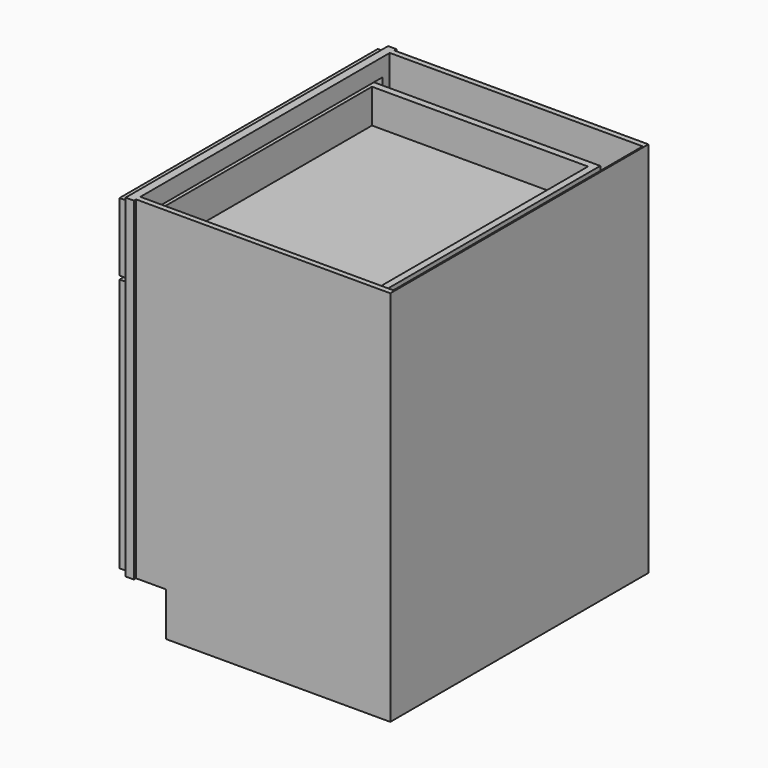
from build123d import *

# Parameters (mm, degrees)
F0_W          = 609.6
F0_H          = 876.3
F1_DEPTH      = 762
F2_W          = 88.9
F2_H          = 101.6
F3_DEPTH      = 762.001
F4_W          = 680.8032786885
F4_H          = 692.15
F5_DEPTH      = 19.05
F6_W          = 590.55
F6_H          = 6.35
F7_DEPTH      = 876.301
F8_W          = 587.375
F8_H          = 723.9
F9_DEPTH      = 733.425
F10_W         = 680.8032786885
F10_H         = 41.275
F11_DEPTH     = 19.05
F12_W         = 374.65
F12_H         = 590.5627
F12_W_2       = 260.35
F12_H_2       = 476.2627
F13_DEPTH     = 19.05
F14_W         = 6.35
F14_H         = 260.35
F15_DEPTH     = 476.2627
F16_SIZE      = 3.175
F17_W         = 749.3
F17_H         = 158.75
F17_W_2       = 635
F17_H_2       = 82.55
F18_DEPTH     = 19.05
F19_W         = 6.35
F19_H         = 635
F20_DEPTH     = 82.55
F21_SIZE      = 3.175
F22_W         = 504.825
F22_H         = 723.9
F23_DEPTH     = 101.6
F24_W         = 660.4
F24_H         = 95.25
F25_DEPTH     = 533.4
F26_T         = 15.875
F26_T3_DEPTH  = 37.249261314
F26_T5_DEPTH  = 37.249261314
F26_T7_DEPTH  = 37.249261314
F26_T9_DEPTH  = 37.249261314
F26_T11_DEPTH = 36.5125
F26_T13_DEPTH = 666.75
F26_T15_DEPTH = 114.3
F26_T17_DEPTH = 127
F26_T19_DEPTH = 692.15
F26_T21_DEPTH = 111.125
F26_T23_DEPTH = 36.5125


# Not quite as in the source:
# - a shell that OpenCascade refuses in one call is made with other operations: the cavity is built on its own and cut out


with BuildPart() as f1:
    # F0 (on Front) → F1 (new body)
    with BuildSketch(Plane.XZ):
        Rectangle(F0_W, F0_H)
    extrude(amount=-F1_DEPTH)

    # F2 (on face) → F3 (cut, through all)
    with BuildSketch(Plane.XZ):
        with Locations((-260.35, -387.35)):
            Rectangle(F2_W, F2_H)
    extrude(amount=-F3_DEPTH, mode=Mode.SUBTRACT)

    # F4 (on face) → F5 (cut)
    with BuildSketch(Plane(origin=(-304.8, 0, 0), x_dir=(0, -1, 0), z_dir=(-1, 0, 0))):
        with Locations((-381, 50.8)):
            Rectangle(F4_W, F4_H)
    extrude(amount=-F5_DEPTH, mode=Mode.SUBTRACT)

    # F6 (on face) → F7 (cut, through all)
    with BuildSketch(Plane.XY.offset(438.15)):
        with Locations((9.525, 758.825)):
            Rectangle(F6_W, F6_H)
        with Locations((9.525, 3.175)):
            Rectangle(F6_W, F6_H)
    extrude(amount=-F7_DEPTH, mode=Mode.SUBTRACT)

    # F8 (on face) → F9 (cut, through all)
    with BuildSketch(Plane.XY.offset(438.15)):
        with Locations((7.9375, 381)):
            Rectangle(F8_W, F8_H)
    extrude(amount=-F9_DEPTH, mode=Mode.SUBTRACT)

    # F10 (on face) → F11 (join, through all)
    with BuildSketch(Plane(origin=(-304.8, 0, 0), x_dir=(0, -1, 0), z_dir=(-1, 0, 0))):
        with Locations((-381, 265.1125)):
            Rectangle(F10_W, F10_H)
    extrude(amount=-F11_DEPTH)

    # F22 (on face) → F23 (cut)
    with BuildSketch(Plane(origin=(0, 0, -438.15), x_dir=(1, 0, 0), z_dir=(0, 0, -1))):
        with Locations((49.2125, -381)):
            Rectangle(F22_W, F22_H)
    extrude(amount=-F23_DEPTH, mode=Mode.SUBTRACT)


with BuildPart() as f13:
    # F12 (on face) → F13 (new body)
    with BuildSketch(Plane(origin=(-304.8, 0, 0), x_dir=(0, -1, 0), z_dir=(-1, 0, 0))):
        with Locations((-568.325, -33.33115)):
            Rectangle(F12_W, F12_H)
        with Locations((-568.325, -33.33115)):
            Rectangle(F12_W_2, F12_H_2, mode=Mode.SUBTRACT)
    extrude(amount=F13_DEPTH)

    # F14 (on face) → F15 (join, through all)
    with BuildSketch(Plane.XY.offset(-271.4625)):
        with Locations((-312.7375, 568.325)):
            Rectangle(F14_W, F14_H)
    extrude(amount=F15_DEPTH)

    # F16
    f16_edges = [f13.edges().sort_by_distance(p)[0] for p in [
        (-323.85, 698.5, -33.33115),
        (-323.85, 568.325, -271.4625),
        (-323.85, 438.15, -33.33115),
        (-323.85, 568.325, 204.8002),
    ]]
    chamfer(f16_edges, length=F16_SIZE)


with BuildPart() as f18:
    # F17 (on face) → F18 (new body)
    with BuildSketch(Plane(origin=(-304.8, 0, 0), x_dir=(0, -1, 0), z_dir=(-1, 0, 0))):
        with Locations((-381, 349.25)):
            Rectangle(F17_W, F17_H)
        with Locations((-381, 349.25)):
            Rectangle(F17_W_2, F17_H_2, mode=Mode.SUBTRACT)
    extrude(amount=F18_DEPTH)

    # F19 (on face) → F20 (join, through all)
    with BuildSketch(Plane.XY.offset(307.975)):
        with Locations((-312.7375, 381)):
            Rectangle(F19_W, F19_H)
    extrude(amount=F20_DEPTH)

    # F21
    f21_edges = [f18.edges().sort_by_distance(p)[0] for p in [
        (-323.85, 381, 307.975),
        (-323.85, 698.5, 349.25),
        (-323.85, 381, 390.525),
        (-323.85, 63.5, 349.25),
    ]]
    chamfer(f21_edges, length=F21_SIZE)

    # F24 (on face) → F25 (join)
    with BuildSketch(Plane.YZ.offset(-304.8)):
        with Locations((381, 339.725)):
            Rectangle(F24_W, F24_H)
    extrude(amount=F25_DEPTH)

    # F26: shell of thickness 15.875, made by hand


with BuildPart() as f26_core1:
    # F26_t2: copy of F18
    add(f18.part)

    # the walls: a layer under each face that stays
    f26_faces = [f26_core1.faces().sort_by_distance(p)[0] for p in [
        (-323.85, 630.7666666667, 296.3333333333),
        (-322.2625, 381, 306.3875),
        (-322.2625, 61.9125, 349.25),
        (-322.2625, 700.0875, 349.25),
        (-322.2625, 381, 392.1125),
        (-314.325, 381, 428.625),
        (-314.325, 755.65, 349.25),
        (-314.325, 381, 269.875),
        (-314.325, 6.35, 349.25),
        (-318.29375, 381, 307.975),
        (-318.29375, 63.5, 349.25),
        (-318.29375, 698.5, 349.25),
        (-318.29375, 381, 390.525),
        (-304.8, 630.7666666667, 402.1666666667),
        (-315.9125, 381, 349.25),
        (-38.1, 711.2, 339.725),
        (-38.1, 381, 292.1),
        (-38.1, 50.8, 339.725),
        (-307.18125, 63.5, 349.25),
        (-307.18125, 381, 390.525),
        (-307.18125, 698.5, 349.25),
        (-304.8, 381, 347.6625),
        (228.6, 381, 339.725),
        (-307.18125, 381, 307.975),
        (-309.5625, 381, 349.25),
    ]]
    thicken(f26_faces, amount=-F26_T, mode=Mode.SUBTRACT)

    # F26_s4 → F26_t3 (cut)
    with BuildSketch(Plane(origin=(4.5928978099, 4.5928978099, 4.5928978099), x_dir=(-0.7071067812, 0.7071067812, 0), z_dir=(0.5773502692, 0.5773502692, 0.5773502692))):
        Polygon((271.8908726623, 356.5892701441), (263.7152476623, 342.7036353262), (255.7777476623, 347.2863530879), (255.7777476623, 356.4517886113), align=None)
    extrude(amount=F26_T3_DEPTH, mode=Mode.SUBTRACT)

    # F26_s6 → F26_t5 (cut)
    with BuildSketch(Plane(origin=(-249.4071021901, 249.40710219, -249.4071021901), x_dir=(0.7071067812, 0.7071067812, 0), z_dir=(0.5773502692, -0.5773502692, 0.5773502692))):
        Polygon((266.9244946018, 667.6744674776), (275.1001196018, 653.7888326596), (283.0376196018, 658.3715504213), (283.0376196018, 667.5369859447), align=None)
    extrude(amount=F26_T5_DEPTH, mode=Mode.SUBTRACT)

    # F26_s8 → F26_t7 (cut)
    with BuildSketch(Plane(origin=(-228.2404355234, -228.2404355234, 228.2404355234), x_dir=(-0.7071067812, 0.7071067812, 0), z_dir=(0.5773502692, 0.5773502692, -0.5773502692))):
        Polygon((271.8908726623, 213.7335916339), (255.7777476623, 213.8710731668), (255.7777476623, 223.0365086901), (263.7152476623, 227.6192264518), align=None)
    extrude(amount=F26_T7_DEPTH, mode=Mode.SUBTRACT)

    # F26_s10 → F26_t9 (cut)
    with BuildSketch(Plane(origin=(-482.2404355234, 482.2404355234, 482.2404355234), x_dir=(0.7071067812, 0.7071067812, 0), z_dir=(0.5773502692, -0.5773502692, -0.5773502692))):
        Polygon((266.9244946018, -97.3516056996), (283.0376196018, -97.2141241667), (283.0376196018, -88.0486886433), (275.1001196018, -83.4659708816), align=None)
    extrude(amount=F26_T9_DEPTH, mode=Mode.SUBTRACT)

    # F26_s12 → F26_t11 (cut)
    with BuildSketch(Plane.YZ.offset(-336.55)):
        Polygon((698.34125, 308.13375), (698.5, 292.1), (714.375, 292.1), (714.375, 307.975), align=None)
        Polygon((63.65875, 308.13375), (63.5, 292.1), (47.625, 292.1), (47.625, 307.975), align=None)
        Polygon((63.65875, 390.36625), (47.625, 390.525), (47.625, 406.4), (63.5, 406.4), align=None)
        Polygon((698.34125, 390.36625), (714.375, 390.525), (714.375, 406.4), (698.5, 406.4), align=None)
    extrude(amount=F26_T11_DEPTH, mode=Mode.SUBTRACT)

    # F26_s14 → F26_t13 (cut)
    with BuildSketch(Plane.XZ.offset(-714.375)):
        Polygon((-316.07125, 308.13375), (-315.9125, 292.1), (-300.0375, 292.1), (-300.0375, 307.975), align=None)
        Polygon((-316.07125, 390.36625), (-315.9125, 406.4), (-300.0375, 406.4), (-300.0375, 390.525), align=None)
        Polygon((-309.40375, 390.36625), (-309.5625, 406.4), (-325.4375, 406.4), (-325.4375, 390.525), align=None)
        Polygon((-304.95875, 308.13375), (-288.925, 307.975), (-288.925, 292.1), (-304.8, 292.1), align=None)
        Polygon((-309.40375, 308.13375), (-309.5625, 292.1), (-325.4375, 292.1), (-325.4375, 307.975), align=None)
    extrude(amount=F26_T13_DEPTH, mode=Mode.SUBTRACT)

    # F26_s16 → F26_t15 (cut)
    with BuildSketch(Plane.XY.offset(292.1)):
        Polygon((-316.07125, 63.65875), (-315.9125, 47.625), (-300.0375, 47.625), (-300.0375, 63.5), align=None)
        Polygon((-316.07125, 698.34125), (-315.9125, 714.375), (-300.0375, 714.375), (-300.0375, 698.5), align=None)
        Polygon((-309.40375, 63.65875), (-309.5625, 47.625), (-325.4375, 47.625), (-325.4375, 63.5), align=None)
        Polygon((-309.40375, 698.34125), (-309.5625, 714.375), (-325.4375, 714.375), (-325.4375, 698.5), align=None)
    extrude(amount=F26_T15_DEPTH, mode=Mode.SUBTRACT)

    # F26_s18 → F26_t17 (cut)
    with BuildSketch(Plane.XY.offset(276.225)):
        Polygon((-304.64125, 711.35875), (-320.675, 711.2), (-320.675, 695.325), (-304.8, 695.325), align=None)
        Polygon((-304.64125, 50.64125), (-320.675, 50.8), (-320.675, 66.675), (-304.8, 66.675), align=None)
    extrude(amount=F26_T17_DEPTH, mode=Mode.SUBTRACT)

    # F26_s20 → F26_t19 (cut)
    with BuildSketch(Plane.XZ.offset(-727.075)):
        Polygon((-304.64125, 291.94125), (-320.675, 292.1), (-320.675, 307.975), (-304.8, 307.975), align=None)
    extrude(amount=F26_T19_DEPTH, mode=Mode.SUBTRACT)

    # F26_s22 → F26_t21 (cut)
    with BuildSketch(Plane.XY.offset(292.1)):
        Polygon((-304.95875, 63.65875), (-304.8, 47.625), (-288.925, 47.625), (-288.925, 63.5), align=None)
        Polygon((-304.95875, 698.34125), (-304.8, 714.375), (-288.925, 714.375), (-288.925, 698.5), align=None)
    extrude(amount=F26_T21_DEPTH, mode=Mode.SUBTRACT)

    # F26_s24 → F26_t23 (cut)
    with BuildSketch(Plane.YZ.offset(-325.4375)):
        Polygon((63.65875, 308.13375), (47.625, 307.975), (47.625, 292.1), (63.5, 292.1), align=None)
        Polygon((63.65875, 390.36625), (47.625, 390.525), (47.625, 406.4), (63.5, 406.4), align=None)
        Polygon((698.34125, 390.36625), (698.5, 406.4), (714.375, 406.4), (714.375, 390.525), align=None)
        Polygon((698.34125, 308.13375), (714.375, 307.975), (714.375, 292.1), (698.5, 292.1), align=None)
    extrude(amount=F26_T23_DEPTH, mode=Mode.SUBTRACT)


with BuildPart() as f18_1:
    add(f18.part)

    # what is left inside the walls is the cavity
    f26_cavity = [f26_core1.part.solids().sort_by_distance(p)[0] for p in [
        (45.508333, 381, 308.13375),
    ]]
    add(f26_cavity, mode=Mode.SUBTRACT)


with BuildPart() as f27_1:
    # F27: instance of F13
    add(f13.part.mirror(Plane(origin=(-314.325, 381, -33.33115), x_dir=(1, 0, 0), z_dir=(0, -1, 0))))


solid = Compound([f1.part, f13.part, f18_1.part, f27_1.part])
